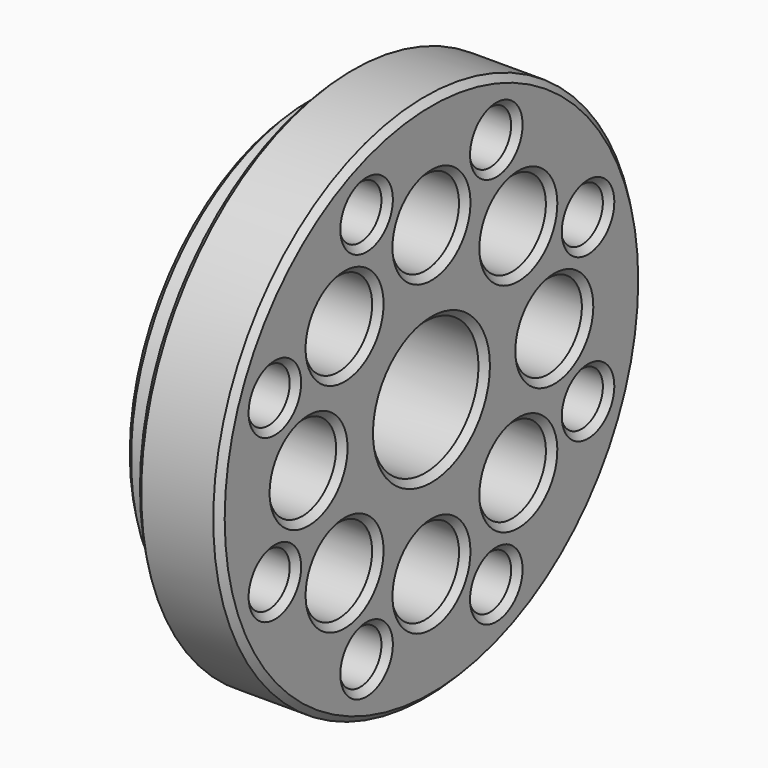
from build123d import *

# Parameters (mm, degrees)
F0_R             = 26.924
F1_DEPTH         = 5.08
F2_R             = 31.75
F3_DEPTH         = 10.16
F4_R             = 8.001
F5_DEPTH         = 15.241
F6_SIZE          = 0.762
F7_R             = 5.08
F8_DEPTH         = 15.241
F8_COPIES_COUNT  = 8
F9_R             = 3.175
F10_DEPTH        = 7.62
F10_COPIES_COUNT = 8
F11_SIZE         = 0.762


# Not quite as in the source:
# - a pattern or mirror of a feature is missing from the dataset's text; its kind, count and spacing are read off the source's solid


with BuildPart() as f1:
    # F0 (on Right) → F1 (new body)
    with BuildSketch(Plane.YZ):
        Circle(F0_R)
    extrude(amount=-F1_DEPTH)

    # F2 (on face) → F3 (join)
    with BuildSketch(Plane.YZ):
        Circle(F2_R)
    extrude(amount=F3_DEPTH)

    # F4 (on face) → F5 (cut, through all)
    with BuildSketch(Plane.YZ.offset(10.16)):
        Circle(F4_R)
    extrude(amount=-F5_DEPTH, mode=Mode.SUBTRACT)

    # F6
    f6_edges = [f1.edges().sort_by_distance(p)[0] for p in [
        (10.16, -8.001, 0),
        (10.16, -31.75, 0),
        (0, -31.75, 0),
        (-5.08, -26.924, 0),
        (-5.08, -8.001, 0),
    ]]
    chamfer(f6_edges, length=F6_SIZE)

    # F7 (on face) → F8 (cut, through all)
    with BuildSketch(Plane(origin=(-5.08, 0, 0), x_dir=(0, -1, 0), z_dir=(-1, 0, 0))):
        with Locations((0, 18.415)):
            Circle(F7_R)
    f8 = extrude(amount=-F8_DEPTH, mode=Mode.SUBTRACT)

    # F8_copies: F8 ×8 about axis
    f8_copies_axis = Axis((0, 0, 0), (1, 0, 0))
    for i in range(1, F8_COPIES_COUNT):
        add(f8.rotate(f8_copies_axis, i * 360 / F8_COPIES_COUNT), mode=Mode.SUBTRACT)

    # F9 (on face) → F10 (cut)
    with BuildSketch(Plane.YZ.offset(10.16)):
        with Locations((-9.7201591821, 23.4665401258)):
            Circle(F9_R)
    f10 = extrude(amount=-F10_DEPTH, mode=Mode.SUBTRACT)

    # F10_copies: F10 ×8 about axis
    f10_copies_axis = Axis((0, 0, 0), (1, 0, 0))
    for i in range(1, F10_COPIES_COUNT):
        add(f10.rotate(f10_copies_axis, i * 360 / F10_COPIES_COUNT), mode=Mode.SUBTRACT)

    # F11
    f11_edges = [f1.edges().sort_by_distance(p)[0] for p in [
        (10.16, -12.895159, 23.46654),
        (10.16, 5.08, 18.415),
        (-5.08, 5.08, 18.415),
        (10.16, -7.475095, -25.711604),
        (10.16, -23.46654, -12.895159),
        (10.16, -16.613474, -9.429269),
        (10.16, 12.895159, -23.46654),
        (10.16, -5.08, -18.415),
        (10.16, 9.429269, -16.613474),
        (10.16, 25.711604, -7.475095),
        (10.16, 18.415, -5.08),
        (10.16, -18.415, 5.08),
        (10.16, -25.711604, 7.475095),
        (10.16, -9.429269, 16.613474),
        (10.16, 16.613474, 9.429269),
        (10.16, 23.46654, 12.895159),
        (10.16, 7.475095, 25.711604),
        (-5.08, -16.613474, -9.429269),
        (-5.08, -5.08, -18.415),
        (-5.08, 9.429269, -16.613474),
        (-5.08, 18.415, -5.08),
        (-5.08, -18.415, 5.08),
        (-5.08, -9.429269, 16.613474),
        (-5.08, 16.613474, 9.429269),
    ]]
    chamfer(f11_edges, length=F11_SIZE)


solid = f1.part
